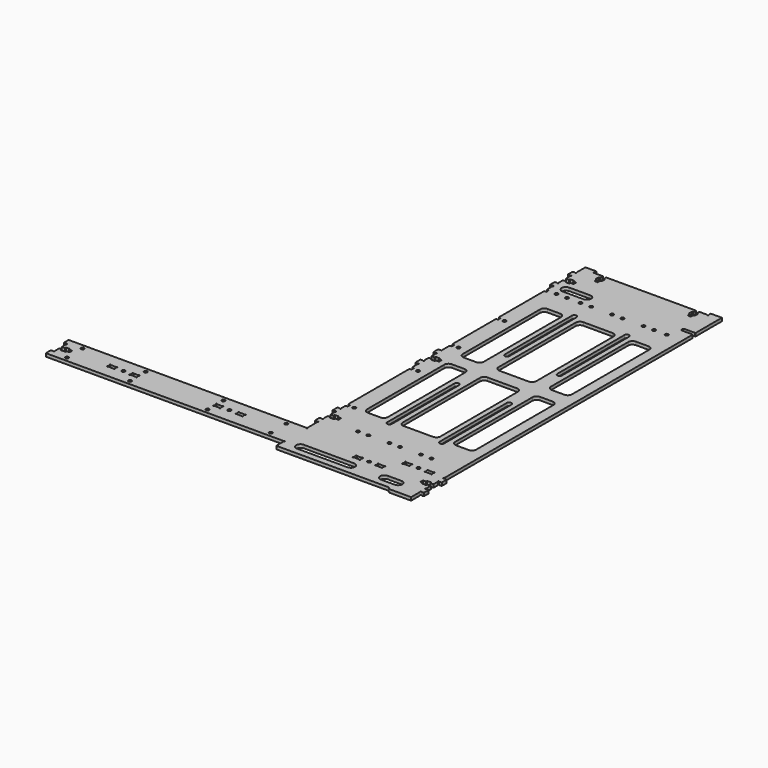
from build123d import *

# Parameters (mm, degrees)
F0_R     = 1.55
F0_R_2   = 1.6
F1_DEPTH = 3


# Not quite as in the source:
# - ends of sketch curves that miss each other by under 0.0002 mm in the source are joined


with BuildPart() as f1:
    # F0 (on Top) → F1 (new body)
    with BuildSketch(Plane.XY):
        with BuildLine():
            ThreePointArc((46.5670159066, -169.5027439461), (47.3535809076, -169.3991911264), (47.2500302369, -170.1857564104))
            ThreePointArc((47.2500302369, -170.1857564104), (47.0670190274, -170.368768469), (47.000032, -170.618767))
            Line((47.000032, -170.618767), (47.000029, -179.152731))
            Line((47.000029, -179.152731), (153.172029, -179.152731))
            ThreePointArc((153.172029, -179.152731), (153.9371645907, -179.3050534338), (154.5858130624, -179.7385159376))
            Line((154.5858130624, -179.7385159376), (155.414245, -180.566946))
            ThreePointArc((155.414245, -180.566946), (156.0630911152, -181.0004904709), (156.828457, -181.152731))
            Line((156.828457, -181.152731), (176.999999, -181.152731))
            Line((176.999999, -181.152731), (176.999998, -170.618767))
            ThreePointArc((176.999998, -170.618767), (176.9330110061, -170.368767527), (176.7499990539, -170.1857549066))
            ThreePointArc((176.7499990539, -170.1857549066), (176.6464475753, -169.3991886435), (177.4330134594, -169.5027443121))
            ThreePointArc((177.4330134594, -169.5027443121), (177.616026152, -169.6857567896), (177.866026, -169.752744))
            Line((177.866026, -169.752744), (179.500053, -169.752747))
            ThreePointArc((179.500053, -169.752747), (179.8536063906, -169.6063003906), (180.000053, -169.252747))
            Line((180.000053, -169.252747), (180.000053, -164.252749))
            ThreePointArc((180.000053, -164.252749), (179.8536063906, -163.8991956094), (179.500053, -163.752749))
            Line((179.500053, -163.752749), (177.866024, -163.752749))
            ThreePointArc((177.866024, -163.752749), (177.616024527, -163.8197359939), (177.4330119066, -164.0027479461))
            ThreePointArc((177.4330119066, -164.0027479461), (176.6464456435, -164.1062994247), (176.7500013121, -163.3197335406))
            ThreePointArc((176.7500013121, -163.3197335406), (176.9330137896, -163.136720848), (177.000001, -162.886721))
            Line((177.000001, -162.886721), (177.000001, -157.752727))
            Line((177.000001, -157.752727), (174.000029, -157.752727))
            Line((174.000029, -157.752727), (174.000029, -159.027722))
            Line((174.000029, -159.027722), (170.000001, -159.027722))
            Line((170.000001, -159.027722), (170.000001, -157.752727))
            Line((170.000001, -157.752727), (167.000001, -157.752727))
            Line((167.000001, -157.752727), (167.000001, -154.552716))
            Line((167.000001, -154.552716), (170.000001, -154.552716))
            Line((170.000001, -154.552716), (170.000001, -153.277722))
            Line((170.000001, -153.277722), (174.000029, -153.277722))
            Line((174.000029, -153.277722), (174.000029, -154.552716))
            Line((174.000029, -154.552716), (177.000001, -154.552716))
            Line((177.000001, -154.552716), (176.999998, -149.418751))
            ThreePointArc((176.999998, -149.418751), (176.9330110061, -149.168751527), (176.7499990539, -148.9857389066))
            ThreePointArc((176.7499990539, -148.9857389066), (176.6464483986, -148.1991728203), (177.4330137764, -148.3027271291))
            ThreePointArc((177.4330137764, -148.3027271291), (177.616026152, -148.4857397896), (177.866026, -148.552727))
            Line((177.866026, -148.552727), (179.500053, -148.55273))
            ThreePointArc((179.500053, -148.55273), (179.8536063906, -148.4062833906), (180.000053, -148.05273))
            Line((180.000053, -148.05273), (180.000053, -143.052733))
            ThreePointArc((180.000053, -143.052733), (179.8536063906, -142.6991796094), (179.500053, -142.552733))
            Line((179.500053, -142.552733), (177.866024, -142.552733))
            ThreePointArc((177.866024, -142.552733), (177.616024527, -142.6197199939), (177.4330119066, -142.8027319461))
            ThreePointArc((177.4330119066, -142.8027319461), (176.6464456435, -142.9062834247), (176.7500013121, -142.1197175406))
            ThreePointArc((176.7500013121, -142.1197175406), (176.9330137896, -141.936704848), (177.000001, -141.686705))
            Line((177.000001, -141.686705), (176.999999, 153.897269))
            Line((176.999999, 153.897269), (176.749999, 154.147269))
            Line((176.749999, 154.147269), (167, 154.147269))
            ThreePointArc((167, 154.147269), (165.4, 155.747269), (167, 157.347269))
            Line((167, 157.347269), (176.749999, 157.347269))
            Line((176.749999, 157.347269), (176.999999, 157.597269))
            Line((176.999999, 157.597269), (176.999999, 188.846999))
            Line((176.999999, 188.846999), (166.349997, 188.846999))
            Line((166.349997, 188.846999), (166.349997, 186.612952))
            ThreePointArc((166.349997, 186.612952), (166.4169843354, 186.3629519355), (166.5999971291, 186.1799392236))
            ThreePointArc((166.5999971291, 186.1799392236), (166.7035498736, 185.3933740924), (165.9169845896, 185.4969247631))
            ThreePointArc((165.9169845896, 185.4969247631), (165.7340559469, 185.6801182191), (165.484029, 185.7472689345))
            Line((165.484029, 185.7472689345), (157.950002, 185.747269))
            Line((157.950002, 185.747269), (157.950002, 182.746955))
            Line((157.950002, 182.746955), (159.224997, 182.746955))
            Line((159.224997, 182.746955), (159.224997, 178.746927))
            Line((159.224997, 178.746927), (157.950002, 178.746927))
            Line((157.950002, 178.746927), (157.950002, 175.746927))
            Line((157.950002, 175.746927), (154.749991, 175.746927))
            Line((154.749991, 175.746927), (154.749991, 178.746927))
            Line((154.749991, 178.746927), (153.474997, 178.746927))
            Line((153.474997, 178.746927), (153.474997, 182.746955))
            Line((153.474997, 182.746955), (154.749991, 182.746955))
            Line((154.749991, 182.746955), (154.749991, 185.746919))
            Line((154.749991, 185.746919), (69.250034, 185.747224))
            Line((69.250034, 185.747224), (69.250034, 182.747252))
            Line((69.250034, 182.747252), (70.525028, 182.747252))
            Line((70.525028, 182.747252), (70.525028, 178.747224))
            Line((70.525028, 178.747224), (69.250034, 178.747224))
            Line((69.250034, 178.747224), (69.250034, 175.747224))
            Line((69.250034, 175.747224), (66.050023, 175.747224))
            Line((66.050023, 175.747224), (66.050023, 178.747224))
            Line((66.050023, 178.747224), (64.775028, 178.747224))
            Line((64.775028, 178.747224), (64.775028, 182.747252))
            Line((64.775028, 182.747252), (66.050023, 182.747252))
            Line((66.050023, 182.747252), (66.050023, 185.747224))
            Line((66.050023, 185.747224), (58.516052, 185.747221))
            ThreePointArc((58.516052, 185.747221), (58.266052527, 185.6802340061), (58.0830399066, 185.4972220539))
            ThreePointArc((58.0830399066, 185.4972220539), (57.2964738203, 185.3936713986), (57.4000281291, 186.1802367764))
            ThreePointArc((57.4000281291, 186.1802367764), (57.5830407896, 186.363249152), (57.650028, 186.613249))
            Line((57.650028, 186.613249), (57.650028, 188.847296))
            Line((57.650028, 188.847296), (47.000029, 188.847296))
            Line((47.000029, 188.847296), (47.000029, 178.313296))
            ThreePointArc((47.000029, 178.313296), (47.0670163354, 178.0632959355), (47.2500291291, 177.8802832236))
            ThreePointArc((47.2500291291, 177.8802832236), (47.3535818736, 177.0937180924), (46.5670165896, 177.1972687631))
            ThreePointArc((46.5670165896, 177.1972687631), (46.384004098, 177.3802802226), (46.134005, 177.447267))
            Line((46.134005, 177.447267), (44.499977, 177.447267))
            ThreePointArc((44.499977, 177.447267), (44.1464236094, 177.3008203906), (43.999977, 176.947267))
            Line((43.999977, 176.947267), (43.999977, 171.94727))
            ThreePointArc((43.999977, 171.94727), (44.1464236094, 171.5937166094), (44.499977, 171.44727))
            Line((44.499977, 171.44727), (46.134003, 171.447273))
            ThreePointArc((46.134003, 171.447273), (46.3840030645, 171.5142603354), (46.5670157764, 171.6972731291))
            ThreePointArc((46.5670157764, 171.6972731291), (47.3535809076, 171.8008258736), (47.2500302369, 171.0142605896))
            ThreePointArc((47.2500302369, 171.0142605896), (47.0670187774, 170.831248098), (47.000032, 170.581249))
            Line((47.000032, 170.581249), (47.000029, 165.447284))
            Line((47.000029, 165.447284), (50.000001, 165.447284))
            Line((50.000001, 165.447284), (50.000001, 166.722279))
            Line((50.000001, 166.722279), (54.000029, 166.722279))
            Line((54.000029, 166.722279), (54.000029, 165.447284))
            Line((54.000029, 165.447284), (57.000029, 165.447284))
            Line((57.000029, 165.447284), (57.000029, 162.247273))
            Line((57.000029, 162.247273), (54.000029, 162.247273))
            Line((54.000029, 162.247273), (54.000029, 160.972279))
            Line((54.000029, 160.972279), (50.000001, 160.972279))
            Line((50.000001, 160.972279), (50.000001, 162.247273))
            Line((50.000001, 162.247273), (47.000029, 162.247273))
            Line((47.000029, 162.247273), (47.000029, 157.113279))
            ThreePointArc((47.000029, 157.113279), (47.0670163354, 156.8632789355), (47.2500291291, 156.6802662236))
            ThreePointArc((47.2500291291, 156.6802662236), (47.3535825674, 155.8936997862), (46.5670164736, 155.9972526961))
            ThreePointArc((46.5670164736, 155.9972526961), (46.384004098, 156.1802642226), (46.134005, 156.247251))
            Line((46.134005, 156.247251), (44.499977, 156.247251))
            ThreePointArc((44.499977, 156.247251), (44.1464236094, 156.1008043906), (43.999977, 155.747251))
            Line((43.999977, 155.747251), (43.999977, 150.747254))
            ThreePointArc((43.999977, 150.747254), (44.1464236094, 150.3937006094), (44.499977, 150.247254))
            Line((44.499977, 150.247254), (46.134003, 150.247257))
            ThreePointArc((46.134003, 150.247257), (46.3840030645, 150.3142443354), (46.5670157764, 150.4972571291))
            ThreePointArc((46.5670157764, 150.4972571291), (47.3535809076, 150.6008098736), (47.2500302369, 149.8142445896))
            ThreePointArc((47.2500302369, 149.8142445896), (47.0670187774, 149.631232098), (47.000032, 149.381233))
            Line((47.000032, 149.381233), (47.000002, 143.347269))
            Line((47.000002, 143.347269), (47.499999, 142.847269))
            Line((47.499999, 142.847269), (48.999999, 142.847269))
            Line((48.999999, 142.847269), (48.999999, 139.847269))
            Line((48.999999, 139.847269), (47.499999, 139.847269))
            Line((47.499999, 139.847269), (46.999999, 139.347269))
            Line((46.999999, 139.347269), (46.999999, 85.847269))
            Line((46.999999, 85.847269), (47.499999, 85.347269))
            Line((47.499999, 85.347269), (48.999999, 85.347269))
            Line((48.999999, 85.347269), (48.999999, 82.347269))
            Line((48.999999, 82.347269), (47.499999, 82.347269))
            Line((47.499999, 82.347269), (46.999999, 81.847269))
            Line((46.999999, 81.847269), (46.999999, 30.847269))
            Line((46.999999, 30.847269), (47.499999, 30.347269))
            Line((47.499999, 30.347269), (48.999999, 30.347269))
            Line((48.999999, 30.347269), (48.999999, 27.347269))
            Line((48.999999, 27.347269), (47.499999, 27.347269))
            Line((47.499999, 27.347269), (47.000001, 26.847269))
            Line((47.000001, 26.847269), (47.000029, 18.313299))
            ThreePointArc((47.000029, 18.313299), (47.0670163354, 18.0632989355), (47.2500291291, 17.8802862236))
            ThreePointArc((47.2500291291, 17.8802862236), (47.3535825674, 17.0937197862), (46.5670164736, 17.1972726961))
            ThreePointArc((46.5670164736, 17.1972726961), (46.384004098, 17.3802842226), (46.134005, 17.447271))
            Line((46.134005, 17.447271), (44.499977, 17.447271))
            ThreePointArc((44.499977, 17.447271), (44.1464236094, 17.3008243906), (43.999977, 16.947271))
            Line((43.999977, 16.947271), (43.999977, 11.947273))
            ThreePointArc((43.999977, 11.947273), (44.1464236094, 11.5937196094), (44.499977, 11.447273))
            Line((44.499977, 11.447273), (46.134003, 11.447276))
            ThreePointArc((46.134003, 11.447276), (46.3840030645, 11.5142633354), (46.5670157764, 11.6972761291))
            ThreePointArc((46.5670157764, 11.6972761291), (47.3535809076, 11.8008288736), (47.2500302369, 11.0142635896))
            ThreePointArc((47.2500302369, 11.0142635896), (47.0670190274, 10.831251531), (47.000032, 10.581253))
            Line((47.000032, 10.581253), (47.000029, 5.447288))
            Line((47.000029, 5.447288), (50.000001, 5.447288))
            Line((50.000001, 5.447288), (50.000001, 6.722282))
            Line((50.000001, 6.722282), (54.000029, 6.722282))
            Line((54.000029, 6.722282), (54.000029, 5.447288))
            Line((54.000029, 5.447288), (57.000029, 5.447288))
            Line((57.000029, 5.447288), (57.000029, 2.247277))
            Line((57.000029, 2.247277), (54.000029, 2.247277))
            Line((54.000029, 2.247277), (54.000029, 0.972282))
            Line((54.000029, 0.972282), (50.000001, 0.972282))
            Line((50.000001, 0.972282), (50.000001, 2.247277))
            Line((50.000001, 2.247277), (47.000029, 2.247277))
            Line((47.000029, 2.247277), (47.000029, -2.886717))
            ThreePointArc((47.000029, -2.886717), (47.0670163354, -3.1367170645), (47.2500291291, -3.3197297764))
            ThreePointArc((47.2500291291, -3.3197297764), (47.3535825674, -4.1062962138), (46.5670164736, -4.0027433039))
            ThreePointArc((46.5670164736, -4.0027433039), (46.384004098, -3.8197317774), (46.134005, -3.752745))
            Line((46.134005, -3.752745), (44.499977, -3.752745))
            ThreePointArc((44.499977, -3.752745), (44.1464236094, -3.8991916094), (43.999977, -4.252745))
            Line((43.999977, -4.252745), (43.999977, -9.252743))
            ThreePointArc((43.999977, -9.252743), (44.1464236094, -9.6062963906), (44.499977, -9.752743))
            Line((44.499977, -9.752743), (46.134003, -9.75274))
            ThreePointArc((46.134003, -9.75274), (46.3840030645, -9.6857526646), (46.5670157764, -9.5027398709))
            ThreePointArc((46.5670157764, -9.5027398709), (47.3535809076, -9.3991871264), (47.2500302369, -10.1857524104))
            ThreePointArc((47.2500302369, -10.1857524104), (47.0670190274, -10.368764469), (47.000032, -10.618763))
            Line((47.000032, -10.618763), (47.000001, -17.152731))
            Line((47.000001, -17.152731), (47.499999, -17.652731))
            Line((47.499999, -17.652731), (48.999999, -17.652731))
            Line((48.999999, -17.652731), (48.999999, -20.652731))
            Line((48.999999, -20.652731), (47.499999, -20.652731))
            Line((47.499999, -20.652731), (46.999999, -21.152731))
            Line((46.999999, -21.152731), (46.999999, -93.152731))
            Line((46.999999, -93.152731), (47.499999, -93.652731))
            Line((47.499999, -93.652731), (48.999999, -93.652731))
            Line((48.999999, -93.652731), (48.999999, -96.652731))
            Line((48.999999, -96.652731), (47.499999, -96.652731))
            Line((47.499999, -96.652731), (47.000002, -97.152731))
            Line((47.000002, -97.152731), (47.000029, -101.686705))
            ThreePointArc((47.000029, -101.686705), (47.0670163354, -101.9367050645), (47.2500291291, -102.1197177764))
            ThreePointArc((47.2500291291, -102.1197177764), (47.3535825674, -102.9062842138), (46.5670164736, -102.8027313039))
            ThreePointArc((46.5670164736, -102.8027313039), (46.384004098, -102.6197197774), (46.134005, -102.552733))
            Line((46.134005, -102.552733), (44.499977, -102.552733))
            ThreePointArc((44.499977, -102.552733), (44.1464236094, -102.6991796094), (43.999977, -103.052733))
            Line((43.999977, -103.052733), (43.999977, -108.05273))
            ThreePointArc((43.999977, -108.05273), (44.1464236094, -108.4062833906), (44.499977, -108.55273))
            Line((44.499977, -108.55273), (46.134003, -108.552727))
            ThreePointArc((46.134003, -108.552727), (46.3840030645, -108.4857396646), (46.5670157764, -108.3027268709))
            ThreePointArc((46.5670157764, -108.3027268709), (47.3535809076, -108.1991741264), (47.2500302369, -108.9857394104))
            ThreePointArc((47.2500302369, -108.9857394104), (47.0670187774, -109.168751902), (47.000032, -109.418751))
            Line((47.000032, -109.418751), (47.000029, -114.552716))
            Line((47.000029, -114.552716), (50.000001, -114.552716))
            Line((50.000001, -114.552716), (50.000001, -113.277722))
            Line((50.000001, -113.277722), (54.000029, -113.277722))
            Line((54.000029, -113.277722), (54.000029, -114.552716))
            Line((54.000029, -114.552716), (57.000029, -114.552716))
            Line((57.000029, -114.552716), (57.000029, -117.752727))
            Line((57.000029, -117.752727), (54.000029, -117.752727))
            Line((54.000029, -117.752727), (54.000029, -119.027722))
            Line((54.000029, -119.027722), (50.000001, -119.027722))
            Line((50.000001, -119.027722), (50.000001, -117.752727))
            Line((50.000001, -117.752727), (47.000029, -117.752727))
            Line((47.000029, -117.752727), (47.000029, -122.886721))
            ThreePointArc((47.000029, -122.886721), (47.0670163354, -123.1367210645), (47.2500291291, -123.3197337764))
            ThreePointArc((47.2500291291, -123.3197337764), (47.3535825674, -124.1063002138), (46.5670164736, -124.0027473039))
            ThreePointArc((46.5670164736, -124.0027473039), (46.384004098, -123.8197357774), (46.134005, -123.752749))
            Line((46.134005, -123.752749), (44.499977, -123.752749))
            ThreePointArc((44.499977, -123.752749), (44.1464236094, -123.8991956094), (43.999977, -124.252749))
            Line((43.999977, -124.252749), (43.999977, -129.252747))
            ThreePointArc((43.999977, -129.252747), (44.1464236094, -129.6063003906), (44.499977, -129.752747))
            Line((44.499977, -129.752747), (46.134003, -129.752744))
            ThreePointArc((46.134003, -129.752744), (46.3840030645, -129.6857566646), (46.5670157764, -129.5027438709))
            ThreePointArc((46.5670157764, -129.5027438709), (47.3535809076, -129.3991911264), (47.2500302369, -130.1857564104))
            ThreePointArc((47.2500302369, -130.1857564104), (47.0670190274, -130.368768469), (47.000032, -130.618767))
            Line((47.000032, -130.618767), (47.000029, -141.686705))
            ThreePointArc((47.000029, -141.686705), (47.0670163354, -141.9367050645), (47.2500291291, -142.1197177764))
            ThreePointArc((47.2500291291, -142.1197177764), (47.3535825674, -142.9062842138), (46.5670164736, -142.8027313039))
            ThreePointArc((46.5670164736, -142.8027313039), (46.384004098, -142.6197197774), (46.134005, -142.552733))
            Line((46.134005, -142.552733), (-179.500054, -142.552733))
            ThreePointArc((-179.500054, -142.552733), (-179.8536073906, -142.6991796094), (-180.000054, -143.052733))
            Line((-180.000054, -143.052733), (-180.000054, -148.05273))
            ThreePointArc((-180.000054, -148.05273), (-179.8536073906, -148.4062833906), (-179.500054, -148.55273))
            Line((-179.500054, -148.55273), (-177.866028, -148.552727))
            ThreePointArc((-177.866028, -148.552727), (-177.6160279355, -148.4857396646), (-177.4330152236, -148.3027268709))
            ThreePointArc((-177.4330152236, -148.3027268709), (-176.6464500924, -148.1991741264), (-176.7500007631, -148.9857394104))
            ThreePointArc((-176.7500007631, -148.9857394104), (-176.9330122226, -149.168751902), (-176.999999, -149.418751))
            Line((-176.999999, -149.418751), (-177.000002, -154.552716))
            Line((-177.000002, -154.552716), (-174.00003, -154.552716))
            Line((-174.00003, -154.552716), (-174.00003, -153.277722))
            Line((-174.00003, -153.277722), (-170.000002, -153.277722))
            Line((-170.000002, -153.277722), (-170.000002, -154.552716))
            Line((-170.000002, -154.552716), (-167.000002, -154.552716))
            Line((-167.000002, -154.552716), (-167.000002, -157.752727))
            Line((-167.000002, -157.752727), (-170.000002, -157.752727))
            Line((-170.000002, -157.752727), (-170.000002, -159.027722))
            Line((-170.000002, -159.027722), (-174.00003, -159.027722))
            Line((-174.00003, -159.027722), (-174.00003, -157.752727))
            Line((-174.00003, -157.752727), (-177.000002, -157.752727))
            Line((-177.000002, -157.752727), (-177.000002, -162.886721))
            ThreePointArc((-177.000002, -162.886721), (-176.9330146646, -163.1367210645), (-176.7500018709, -163.3197337764))
            ThreePointArc((-176.7500018709, -163.3197337764), (-176.6464481264, -164.1062999076), (-177.4330140934, -164.0027480539))
            ThreePointArc((-177.4330140934, -164.0027480539), (-177.616026527, -163.8197359939), (-177.866026, -163.752749))
            Line((-177.866026, -163.752749), (-179.500054, -163.752749))
            ThreePointArc((-179.500054, -163.752749), (-179.8536073906, -163.8991956094), (-180.000054, -164.252749))
            Line((-180.000054, -164.252749), (-180.000054, -169.252747))
            ThreePointArc((-180.000054, -169.252747), (-179.8536073906, -169.6063003906), (-179.500054, -169.752747))
            Line((-179.500054, -169.752747), (46.134003, -169.752744))
            ThreePointArc((46.134003, -169.752744), (46.3840030645, -169.6857566646), (46.5670159066, -169.5027439461))
        make_face()
        with Locations((-163.246874, -165.446001)):
            Circle(F0_R, mode=Mode.SUBTRACT)
        with Locations((-163.247001, -146.859431)):
            Circle(F0_R, mode=Mode.SUBTRACT)
        with Locations((-103.246874, -165.446001)):
            Circle(F0_R, mode=Mode.SUBTRACT)
        with BuildLine():
            Line((-124.500035, -155.368743), (-124.500038, -156.93661))
            ThreePointArc((-124.500038, -156.93661), (-124.4330506646, -157.1866100645), (-124.2500378709, -157.3696227764))
            ThreePointArc((-124.2500378709, -157.3696227764), (-124.146483997, -158.1561877782), (-124.9330496604, -158.0526368039))
            ThreePointArc((-124.9330496604, -158.0526368039), (-125.116062902, -157.8696257774), (-125.366062, -157.802639))
            Line((-125.366062, -157.802639), (-129.834011, -157.802639))
            ThreePointArc((-129.834011, -157.802639), (-130.0840110645, -157.8696263354), (-130.2670237764, -158.0526391291))
            ThreePointArc((-130.2670237764, -158.0526391291), (-131.0535889076, -158.1561918736), (-130.9500382369, -157.3696265896))
            ThreePointArc((-130.9500382369, -157.3696265896), (-130.7670267774, -157.186614098), (-130.70004, -156.936615))
            Line((-130.70004, -156.936615), (-130.700037, -155.368745))
            ThreePointArc((-130.700037, -155.368745), (-130.7670240854, -155.1187443685), (-130.9500371291, -154.9357312236))
            ThreePointArc((-130.9500371291, -154.9357312236), (-131.0535896968, -154.1491659156), (-130.2670243396, -154.2527171961))
            ThreePointArc((-130.2670243396, -154.2527171961), (-130.0840122565, -154.4357291311), (-129.834013, -154.502716))
            Line((-129.834013, -154.502716), (-125.366063, -154.502719))
            ThreePointArc((-125.366063, -154.502719), (-125.1160629355, -154.4357316646), (-124.9330502236, -154.2527188709))
            ThreePointArc((-124.9330502236, -154.2527188709), (-124.1464852218, -154.149164997), (-124.2500361961, -154.9357306604))
            ThreePointArc((-124.2500361961, -154.9357306604), (-124.4330480061, -155.118743527), (-124.500035, -155.368743))
        make_face(mode=Mode.SUBTRACT)
        with Locations((-117.000038, -156.152677)):
            Circle(F0_R_2, mode=Mode.SUBTRACT)
        with BuildLine():
            Line((-103.300036, -155.368743), (-103.300039, -156.93661))
            ThreePointArc((-103.300039, -156.93661), (-103.2330516646, -157.1866100645), (-103.0500388709, -157.3696227764))
            ThreePointArc((-103.0500388709, -157.3696227764), (-102.9464838203, -158.1561886014), (-103.7330500934, -158.0526370539))
            ThreePointArc((-103.7330500934, -158.0526370539), (-103.916062902, -157.8696257774), (-104.166062, -157.802639))
            Line((-104.166062, -157.802639), (-108.634012, -157.802639))
            ThreePointArc((-108.634012, -157.802639), (-108.8840114976, -157.8696265854), (-109.0670237764, -158.0526391291))
            ThreePointArc((-109.0670237764, -158.0526391291), (-109.8535889076, -158.1561918736), (-109.7500382369, -157.3696265896))
            ThreePointArc((-109.7500382369, -157.3696265896), (-109.5670267774, -157.186614098), (-109.50004, -156.936615))
            Line((-109.50004, -156.936615), (-109.500037, -155.368745))
            ThreePointArc((-109.500037, -155.368745), (-109.5670240854, -155.1187443685), (-109.7500371291, -154.9357312236))
            ThreePointArc((-109.7500371291, -154.9357312236), (-109.853592003, -154.1491652218), (-109.0670256566, -154.2527173791))
            ThreePointArc((-109.0670256566, -154.2527173791), (-108.8840132565, -154.4357291311), (-108.634014, -154.502716))
            Line((-108.634014, -154.502716), (-104.166064, -154.502719))
            ThreePointArc((-104.166064, -154.502719), (-103.9160639355, -154.4357316646), (-103.7330512236, -154.2527188709))
            ThreePointArc((-103.7330512236, -154.2527188709), (-102.9464862218, -154.149164997), (-103.0500371961, -154.9357306604))
            ThreePointArc((-103.0500371961, -154.9357306604), (-103.2330490061, -155.118743527), (-103.300036, -155.368743))
        make_face(mode=Mode.SUBTRACT)
        with Locations((-103.246874, -146.859478)):
            Circle(F0_R, mode=Mode.SUBTRACT)
        with Locations((-29.246874, -165.446001)):
            Circle(F0_R, mode=Mode.SUBTRACT)
        with BuildLine():
            Line((-23.49992, -155.368788), (-23.499923, -156.936655))
            ThreePointArc((-23.499923, -156.936655), (-23.4329359146, -157.1866546315), (-23.2499228709, -157.3696677764))
            ThreePointArc((-23.2499228709, -157.3696677764), (-23.1463701264, -158.1562329076), (-23.9329354104, -158.0526822369))
            ThreePointArc((-23.9329354104, -158.0526822369), (-24.115947902, -157.8696707774), (-24.365947, -157.802684))
            Line((-24.365947, -157.802684), (-28.833896, -157.802684))
            ThreePointArc((-28.833896, -157.802684), (-29.0838962565, -157.8696708689), (-29.2669093434, -158.0526833791))
            ThreePointArc((-29.2669093434, -158.0526833791), (-30.0534750844, -158.1562366968), (-29.9499238039, -157.3696713396))
            ThreePointArc((-29.9499238039, -157.3696713396), (-29.7669119939, -157.186658473), (-29.699925, -156.936659))
            Line((-29.699925, -156.936659), (-29.699922, -155.368789))
            ThreePointArc((-29.699922, -155.368789), (-29.7669090854, -155.1187893685), (-29.9499221291, -154.9357762236))
            ThreePointArc((-29.9499221291, -154.9357762236), (-30.053476003, -154.1492112218), (-29.2669103396, -154.2527621961))
            ThreePointArc((-29.2669103396, -154.2527621961), (-29.083897473, -154.4357740061), (-28.833898, -154.502761))
            Line((-28.833898, -154.502761), (-24.365948, -154.502764))
            ThreePointArc((-24.365948, -154.502764), (-24.1159485024, -154.4357764146), (-23.9329362236, -154.2527638709))
            ThreePointArc((-23.9329362236, -154.2527638709), (-23.1463709156, -154.1492103032), (-23.2499221961, -154.9357756604))
            ThreePointArc((-23.2499221961, -154.9357756604), (-23.4329332226, -155.118788902), (-23.49992, -155.368788))
        make_face(mode=Mode.SUBTRACT)
        with Locations((-29.246874, -146.859476)):
            Circle(F0_R, mode=Mode.SUBTRACT)
        with Locations((-15.999923, -156.152721)):
            Circle(F0_R_2, mode=Mode.SUBTRACT)
        with BuildLine():
            Line((-2.299921, -155.368788), (-2.299924, -156.936655))
            ThreePointArc((-2.299924, -156.936655), (-2.2329369146, -157.1866546315), (-2.0499238709, -157.3696677764))
            ThreePointArc((-2.0499238709, -157.3696677764), (-1.9463688203, -158.1562336014), (-2.7329350934, -158.0526820539))
            ThreePointArc((-2.7329350934, -158.0526820539), (-2.915947902, -157.8696707774), (-3.165947, -157.802684))
            Line((-3.165947, -157.802684), (-7.633897, -157.802684))
            ThreePointArc((-7.633897, -157.802684), (-7.8838970645, -157.8696713354), (-8.0669097764, -158.0526841291))
            ThreePointArc((-8.0669097764, -158.0526841291), (-8.8534750844, -158.1562366968), (-8.7499238039, -157.3696713396))
            ThreePointArc((-8.7499238039, -157.3696713396), (-8.5669119939, -157.186658473), (-8.499925, -156.936659))
            Line((-8.499925, -156.936659), (-8.499922, -155.368789))
            ThreePointArc((-8.499922, -155.368789), (-8.5669090854, -155.1187893685), (-8.7499221291, -154.9357762236))
            ThreePointArc((-8.7499221291, -154.9357762236), (-8.8534771797, -154.1492103986), (-8.0669109066, -154.2527619461))
            ThreePointArc((-8.0669109066, -154.2527619461), (-7.883898473, -154.4357740061), (-7.633899, -154.502761))
            Line((-7.633899, -154.502761), (-3.165949, -154.502764))
            ThreePointArc((-3.165949, -154.502764), (-2.9159495024, -154.4357764146), (-2.7329372236, -154.2527638709))
            ThreePointArc((-2.7329372236, -154.2527638709), (-1.9463719156, -154.1492103032), (-2.0499231961, -154.9357756604))
            ThreePointArc((-2.0499231961, -154.9357756604), (-2.2329342226, -155.118788902), (-2.299921, -155.368788))
        make_face(mode=Mode.SUBTRACT)
        with Locations((30.753126, -165.446001)):
            Circle(F0_R, mode=Mode.SUBTRACT)
        with Locations((30.753126, -146.859476)):
            Circle(F0_R, mode=Mode.SUBTRACT)
        with BuildLine():
            Line((110.000029, -173.152731), (62.000029, -173.152731))
            ThreePointArc((62.000029, -173.152731), (58.000029, -169.152731), (62.000029, -165.152731))
            Line((62.000029, -165.152731), (110.000029, -165.152731))
            ThreePointArc((110.000029, -165.152731), (114.000029, -169.152731), (110.000029, -173.152731))
        make_face(mode=Mode.SUBTRACT)
        with Locations((79.999999, -123.152731)):
            Circle(F0_R, mode=Mode.SUBTRACT)
        with Locations((89.999999, -123.152731)):
            Circle(F0_R, mode=Mode.SUBTRACT)
        with Locations((53.999999, -95.152731)):
            Circle(F0_R, mode=Mode.SUBTRACT)
        with BuildLine():
            Line((109.499937, -155.368778), (109.499934, -156.936645))
            ThreePointArc((109.499934, -156.936645), (109.5669209604, -157.186645415), (109.7499336961, -157.3696585264))
            ThreePointArc((109.7499336961, -157.3696585264), (109.8534878736, -158.1562239076), (109.0669219066, -158.0526720539))
            ThreePointArc((109.0669219066, -158.0526720539), (108.883909098, -157.8696607774), (108.63391, -157.802674))
            Line((108.63391, -157.802674), (104.165961, -157.802674))
            ThreePointArc((104.165961, -157.802674), (103.9159609355, -157.8696613354), (103.7329482236, -158.0526741291))
            ThreePointArc((103.7329482236, -158.0526741291), (102.946381963, -158.1562267441), (103.0499335131, -157.3696611566))
            ThreePointArc((103.0499335131, -157.3696611566), (103.2329452226, -157.186649098), (103.299932, -156.93665))
            Line((103.299932, -156.93665), (103.299935, -155.36878))
            ThreePointArc((103.299935, -155.36878), (103.2329480396, -155.118779585), (103.0499353039, -154.9357664736))
            ThreePointArc((103.0499353039, -154.9357664736), (102.9463819497, -154.1492012691), (103.7329474104, -154.2527517631))
            ThreePointArc((103.7329474104, -154.2527517631), (103.915959527, -154.4357640061), (104.165959, -154.502751))
            Line((104.165959, -154.502751), (108.633909, -154.502754))
            ThreePointArc((108.633909, -154.502754), (108.883908848, -154.4357667896), (109.0669215264, -154.2527543039))
            ThreePointArc((109.0669215264, -154.2527543039), (109.8534866014, -154.1491998203), (109.7499358039, -154.9357656604))
            ThreePointArc((109.7499358039, -154.9357656604), (109.5669239939, -155.118778527), (109.499937, -155.368778))
        make_face(mode=Mode.SUBTRACT)
        with Locations((116.999934, -156.152712)):
            Circle(F0_R_2, mode=Mode.SUBTRACT)
        with BuildLine():
            Line((130.699936, -155.368778), (130.699933, -156.936645))
            ThreePointArc((130.699933, -156.936645), (130.7669199604, -157.186645415), (130.9499326961, -157.3696585264))
            ThreePointArc((130.9499326961, -157.3696585264), (131.0534880503, -158.1562247309), (130.2669214736, -158.0526723039))
            ThreePointArc((130.2669214736, -158.0526723039), (130.083909098, -157.8696607774), (129.83391, -157.802674))
            Line((129.83391, -157.802674), (125.36596, -157.802674))
            ThreePointArc((125.36596, -157.802674), (125.1159605024, -157.8696615854), (124.9329482236, -158.0526741291))
            ThreePointArc((124.9329482236, -158.0526741291), (124.146381963, -158.1562267441), (124.2499335131, -157.3696611566))
            ThreePointArc((124.2499335131, -157.3696611566), (124.4329452226, -157.186649098), (124.499932, -156.93665))
            Line((124.499932, -156.93665), (124.499935, -155.36878))
            ThreePointArc((124.499935, -155.36878), (124.4329480396, -155.118779585), (124.2499353039, -154.9357664736))
            ThreePointArc((124.2499353039, -154.9357664736), (124.1463796435, -154.1492005753), (124.9329460934, -154.2527519461))
            ThreePointArc((124.9329460934, -154.2527519461), (125.115958527, -154.4357640061), (125.365958, -154.502751))
            Line((125.365958, -154.502751), (129.833908, -154.502754))
            ThreePointArc((129.833908, -154.502754), (130.083907848, -154.4357667896), (130.2669205264, -154.2527543039))
            ThreePointArc((130.2669205264, -154.2527543039), (131.0534856014, -154.1491998203), (130.9499348039, -154.9357656604))
            ThreePointArc((130.9499348039, -154.9357656604), (130.7669229939, -155.118778527), (130.699936, -155.368778))
        make_face(mode=Mode.SUBTRACT)
        with BuildLine():
            Line((142.000028, -165.152731), (155.000029, -165.152731))
            ThreePointArc((155.000029, -165.152731), (159.000029, -169.152731), (155.000029, -173.152731))
            Line((155.000029, -173.152731), (142.000028, -173.152731))
            ThreePointArc((142.000028, -173.152731), (138.000028, -169.152731), (142.000028, -165.152731))
        make_face(mode=Mode.SUBTRACT)
        with BuildLine():
            Line((144.500002, -140.368797), (144.499999, -141.936664))
            ThreePointArc((144.499999, -141.936664), (144.5669859604, -142.186664415), (144.7499986961, -142.3696775264))
            ThreePointArc((144.7499986961, -142.3696775264), (144.8535531797, -143.1562426014), (144.0669873396, -143.0526918039))
            ThreePointArc((144.0669873396, -143.0526918039), (143.883974473, -142.8696799939), (143.633975, -142.802693))
            Line((143.633975, -142.802693), (139.166026, -142.802693))
            ThreePointArc((139.166026, -142.802693), (138.916025585, -142.8696799604), (138.7330124736, -143.0526926961))
            ThreePointArc((138.7330124736, -143.0526926961), (137.9464473986, -143.1562471797), (138.0499981961, -142.3696813396))
            ThreePointArc((138.0499981961, -142.3696813396), (138.2330100061, -142.186668473), (138.299997, -141.936669))
            Line((138.299997, -141.936669), (138.3, -140.368799))
            ThreePointArc((138.3, -140.368799), (138.2330130396, -140.118798585), (138.0500003039, -139.9357854736))
            ThreePointArc((138.0500003039, -139.9357854736), (137.9464458203, -139.1492203986), (138.7330116604, -139.2527711961))
            ThreePointArc((138.7330116604, -139.2527711961), (138.916024527, -139.4357830061), (139.166024, -139.50277))
            Line((139.166024, -139.50277), (143.633974, -139.502773))
            ThreePointArc((143.633974, -139.502773), (143.883973848, -139.4357857896), (144.0669865264, -139.2527733039))
            ThreePointArc((144.0669865264, -139.2527733039), (144.8535516014, -139.1492188203), (144.7500008039, -139.9357846604))
            ThreePointArc((144.7500008039, -139.9357846604), (144.5669889939, -140.118797527), (144.500002, -140.368797))
        make_face(mode=Mode.SUBTRACT)
        with Locations((151.999999, -141.152731)):
            Circle(F0_R_2, mode=Mode.SUBTRACT)
        with BuildLine():
            Line((165.700001, -140.368797), (165.699998, -141.936664))
            ThreePointArc((165.699998, -141.936664), (165.7669849604, -142.186664415), (165.9499976961, -142.3696775264))
            ThreePointArc((165.9499976961, -142.3696775264), (166.0535533565, -143.1562434247), (165.2669869066, -143.0526920539))
            ThreePointArc((165.2669869066, -143.0526920539), (165.083974473, -142.8696799939), (164.833975, -142.802693))
            Line((164.833975, -142.802693), (160.366025, -142.802693))
            ThreePointArc((160.366025, -142.802693), (160.116025152, -142.8696802104), (159.9330124736, -143.0526926961))
            ThreePointArc((159.9330124736, -143.0526926961), (159.1464473986, -143.1562471797), (159.2499981961, -142.3696813396))
            ThreePointArc((159.2499981961, -142.3696813396), (159.4330100061, -142.186668473), (159.499997, -141.936669))
            Line((159.499997, -141.936669), (159.5, -140.368799))
            ThreePointArc((159.5, -140.368799), (159.4330130396, -140.118798585), (159.2500003039, -139.9357854736))
            ThreePointArc((159.2500003039, -139.9357854736), (159.1464449497, -139.1492192691), (159.9330115264, -139.2527716961))
            ThreePointArc((159.9330115264, -139.2527716961), (160.116023902, -139.4357832226), (160.366023, -139.50277))
            Line((160.366023, -139.50277), (164.833973, -139.502773))
            ThreePointArc((164.833973, -139.502773), (165.083972848, -139.4357857896), (165.2669855264, -139.2527733039))
            ThreePointArc((165.2669855264, -139.2527733039), (166.0535506014, -139.1492188203), (165.9499998039, -139.9357846604))
            ThreePointArc((165.9499998039, -139.9357846604), (165.7669879939, -140.118797527), (165.700001, -140.368797))
        make_face(mode=Mode.SUBTRACT)
        with Locations((109.999999, -123.152731)):
            Circle(F0_R, mode=Mode.SUBTRACT)
        with Locations((119.999999, -123.152731)):
            Circle(F0_R, mode=Mode.SUBTRACT)
        with Locations((139.999999, -123.152731)):
            Circle(F0_R, mode=Mode.SUBTRACT)
        with Locations((149.999999, -123.152731)):
            Circle(F0_R, mode=Mode.SUBTRACT)
        with BuildLine():
            Line((87.799999, -98.152731), (87.799999, -18.152731))
            ThreePointArc((87.799999, -18.152731), (89.999999, -15.952731), (92.199999, -18.152731))
            Line((92.199999, -18.152731), (92.199999, -98.152731))
            ThreePointArc((92.199999, -98.152731), (89.999999, -100.352731), (87.799999, -98.152731))
        make_face(mode=Mode.SUBTRACT)
        with BuildLine():
            Line((66.999969, 4.847269), (78.999969, 4.847269))
            ThreePointArc((78.999969, 4.847269), (81.8283961247, 3.6756961247), (82.999969, 0.847269))
            Line((82.999969, 0.847269), (82.999969, -91.152731))
            ThreePointArc((82.999969, -91.152731), (81.8283961247, -93.9811581247), (78.999969, -95.152731))
            Line((78.999969, -95.152731), (66.999969, -95.152731))
            ThreePointArc((66.999969, -95.152731), (64.1715418753, -93.9811581247), (62.999969, -91.152731))
            Line((62.999969, -91.152731), (62.999969, 0.847269))
            ThreePointArc((62.999969, 0.847269), (64.1715418753, 3.6756961247), (66.999969, 4.847269))
        make_face(mode=Mode.SUBTRACT)
        with Locations((53.999999, -19.152731)):
            Circle(F0_R, mode=Mode.SUBTRACT)
        with BuildLine():
            Line((101.000029, 4.847269), (128.999969, 4.847269))
            ThreePointArc((128.999969, 4.847269), (131.8283961247, 3.6756961247), (132.999969, 0.847269))
            Line((132.999969, 0.847269), (132.999969, -91.152731))
            ThreePointArc((132.999969, -91.152731), (131.8283961247, -93.9811581247), (128.999969, -95.152731))
            Line((128.999969, -95.152731), (101.000029, -95.152731))
            ThreePointArc((101.000029, -95.152731), (98.1716018753, -93.9811581247), (97.000029, -91.152731))
            Line((97.000029, -91.152731), (97.000029, 0.847269))
            ThreePointArc((97.000029, 0.847269), (98.1716018753, 3.6756961247), (101.000029, 4.847269))
        make_face(mode=Mode.SUBTRACT)
        with BuildLine():
            Line((137.799999, -98.152731), (137.799999, -18.152731))
            ThreePointArc((137.799999, -18.152731), (139.999999, -15.952731), (142.199999, -18.152731))
            Line((142.199999, -18.152731), (142.199999, -98.152731))
            ThreePointArc((142.199999, -98.152731), (139.999999, -100.352731), (137.799999, -98.152731))
        make_face(mode=Mode.SUBTRACT)
        with BuildLine():
            Line((147.000029, -91.152731), (147.000029, 0.847269))
            ThreePointArc((147.000029, 0.847269), (148.1716018753, 3.6756961247), (151.000029, 4.847269))
            Line((151.000029, 4.847269), (163.000029, 4.847269))
            ThreePointArc((163.000029, 4.847269), (165.8284561247, 3.6756961247), (167.000029, 0.847269))
            Line((167.000029, 0.847269), (167.000029, -91.152731))
            ThreePointArc((167.000029, -91.152731), (165.8284561247, -93.9811581247), (163.000029, -95.152731))
            Line((163.000029, -95.152731), (151.000029, -95.152731))
            ThreePointArc((151.000029, -95.152731), (148.1716018753, -93.9811581247), (147.000029, -91.152731))
        make_face(mode=Mode.SUBTRACT)
        with Locations((53.999999, 28.847269)):
            Circle(F0_R, mode=Mode.SUBTRACT)
        with BuildLine():
            Line((82.999969, 114.847269), (82.999969, 22.847269))
            ThreePointArc((82.999969, 22.847269), (81.8283961247, 20.0188418753), (78.999969, 18.847269))
            Line((78.999969, 18.847269), (66.999969, 18.847269))
            ThreePointArc((66.999969, 18.847269), (64.1715418753, 20.0188418753), (62.999969, 22.847269))
            Line((62.999969, 22.847269), (62.999969, 114.847269))
            ThreePointArc((62.999969, 114.847269), (64.1715418753, 117.6756961247), (66.999969, 118.847269))
            Line((66.999969, 118.847269), (78.999969, 118.847269))
            ThreePointArc((78.999969, 118.847269), (81.8283961247, 117.6756961247), (82.999969, 114.847269))
        make_face(mode=Mode.SUBTRACT)
        with Locations((53.999999, 83.847269)):
            Circle(F0_R, mode=Mode.SUBTRACT)
        with BuildLine():
            Line((92.199999, 121.847269), (92.199999, 41.847269))
            ThreePointArc((92.199999, 41.847269), (89.999999, 39.647269), (87.799999, 41.847269))
            Line((87.799999, 41.847269), (87.799999, 121.847269))
            ThreePointArc((87.799999, 121.847269), (89.999999, 124.047269), (92.199999, 121.847269))
        make_face(mode=Mode.SUBTRACT)
        with BuildLine():
            Line((132.999969, 114.847269), (132.999969, 22.847269))
            ThreePointArc((132.999969, 22.847269), (131.8283961247, 20.0188418753), (128.999969, 18.847269))
            Line((128.999969, 18.847269), (101.000029, 18.847269))
            ThreePointArc((101.000029, 18.847269), (98.1716018753, 20.0188418753), (97.000029, 22.847269))
            Line((97.000029, 22.847269), (97.000029, 114.847269))
            ThreePointArc((97.000029, 114.847269), (98.1716018753, 117.6756961247), (101.000029, 118.847269))
            Line((101.000029, 118.847269), (128.999969, 118.847269))
            ThreePointArc((128.999969, 118.847269), (131.8283961247, 117.6756961247), (132.999969, 114.847269))
        make_face(mode=Mode.SUBTRACT)
        with BuildLine():
            Line((163.000029, 18.847269), (151.000029, 18.847269))
            ThreePointArc((151.000029, 18.847269), (148.1716018753, 20.0188418753), (147.000029, 22.847269))
            Line((147.000029, 22.847269), (147.000029, 114.847269))
            ThreePointArc((147.000029, 114.847269), (148.1716018753, 117.6756961247), (151.000029, 118.847269))
            Line((151.000029, 118.847269), (163.000029, 118.847269))
            ThreePointArc((163.000029, 118.847269), (165.8284561247, 117.6756961247), (167.000029, 114.847269))
            Line((167.000029, 114.847269), (167.000029, 22.847269))
            ThreePointArc((167.000029, 22.847269), (165.8284561247, 20.0188418753), (163.000029, 18.847269))
        make_face(mode=Mode.SUBTRACT)
        with BuildLine():
            Line((142.199999, 121.847269), (142.199999, 41.847269))
            ThreePointArc((142.199999, 41.847269), (139.999999, 39.647269), (137.799999, 41.847269))
            Line((137.799999, 41.847269), (137.799999, 121.847269))
            ThreePointArc((137.799999, 121.847269), (139.999999, 124.047269), (142.199999, 121.847269))
        make_face(mode=Mode.SUBTRACT)
        with Locations((57.000029, 141.847269)):
            Circle(F0_R, mode=Mode.SUBTRACT)
        with Locations((67.000029, 141.847269)):
            Circle(F0_R, mode=Mode.SUBTRACT)
        with Locations((80.000029, 141.847269)):
            Circle(F0_R, mode=Mode.SUBTRACT)
        with BuildLine():
            Line((77.999999, 147.847269), (57.999999, 147.847269))
            ThreePointArc((57.999999, 147.847269), (53.999999, 151.847269), (57.999999, 155.847269))
            Line((57.999999, 155.847269), (77.999999, 155.847269))
            ThreePointArc((77.999999, 155.847269), (81.999999, 151.847269), (77.999999, 147.847269))
        make_face(mode=Mode.SUBTRACT)
        with Locations((90.000029, 141.847269)):
            Circle(F0_R, mode=Mode.SUBTRACT)
        with Locations((110.000029, 141.847269)):
            Circle(F0_R, mode=Mode.SUBTRACT)
        with Locations((120.000029, 141.847269)):
            Circle(F0_R, mode=Mode.SUBTRACT)
        with Locations((140.000029, 141.847269)):
            Circle(F0_R, mode=Mode.SUBTRACT)
        with Locations((150.000029, 141.847269)):
            Circle(F0_R, mode=Mode.SUBTRACT)
        with Locations((162.000029, 141.847269)):
            Circle(F0_R, mode=Mode.SUBTRACT)
    extrude(amount=F1_DEPTH)


solid = f1.part
